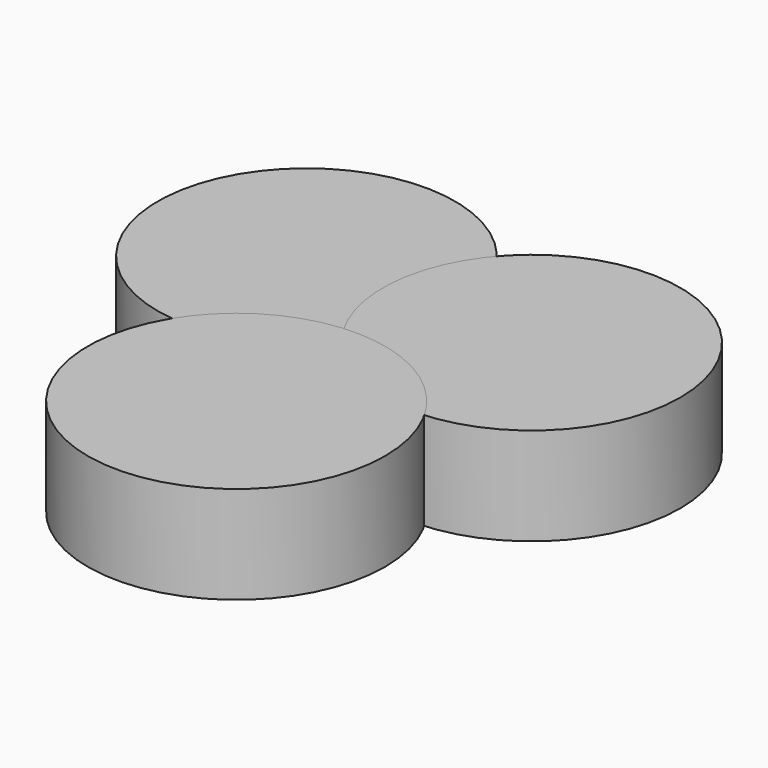
from build123d import *

# Parameters (mm, degrees)
F0_R     = 38.1
F1_DEPTH = 25


# Not quite as in the source:
# - a feature of the source that left no trace in its solid (it failed there, or was rolled back) is left out


with BuildPart() as f1:
    # F0 (on Top) → F1 (new body)
    with BuildSketch(Plane.XY):
        with Locations((-28.6366734654, 28.6366734654)):
            Circle(F0_R)
    extrude(amount=F1_DEPTH)


with BuildPart() as f2_1:
    # F2: copy of F1
    add(f1.part.moved(Location((58.6, -1.1, 0))))


with BuildPart() as f3_1:
    # F3: copy of F1
    add(f1.part.moved(Location((28.3, -57.8, 0))))


solid = Compound([f1.part, f2_1.part, f3_1.part])
